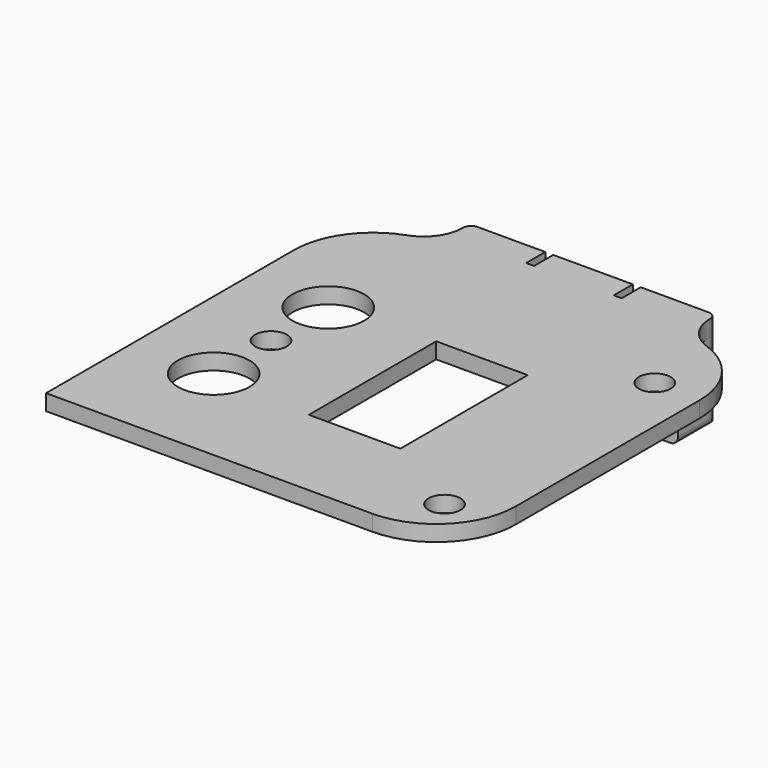
from build123d import *

# Parameters (mm, degrees)
F0_W     = 51
F0_H     = 48
F0_R     = 4.5
F0_R_2   = 2
F0_W_2   = 11.5
F0_H_2   = 20
F1_DEPTH = 2
F3_DEPTH = 6
F4_W     = 1
F4_H     = 12
F5_DEPTH = 3
F6_R     = 5
F7_R     = 0.99999
F8_R     = 10


# Not quite as in the source:
# - a fillet or chamfer is up to 0.001 mm smaller than in the source, because OpenCascade refuses the exact size


with BuildPart() as f1:
    # F0 (on Top) → F1 (new body)
    with BuildSketch(Plane.XY):
        with Locations((25.5, 24)):
            Rectangle(F0_W, F0_H)
        with Locations((10.25, 13.5)):
            Circle(F0_R, mode=Mode.SUBTRACT)
        with Locations((10.25, 22.5)):
            Circle(F0_R_2, mode=Mode.SUBTRACT)
        with Locations((45.25, 6)):
            Circle(F0_R_2, mode=Mode.SUBTRACT)
        with Locations((28.75, 22.5)):
            Rectangle(F0_W_2, F0_H_2, mode=Mode.SUBTRACT)
        with Locations((10.25, 31.5)):
            Circle(F0_R, mode=Mode.SUBTRACT)
        with Locations((45.25, 39)):
            Circle(F0_R_2, mode=Mode.SUBTRACT)
    extrude(amount=F1_DEPTH)

    # F2 (on face) → F3 (join)
    with BuildSketch(Plane(origin=(0, 48, 0), x_dir=(-1, 0, 0), z_dir=(0, 1, 0))):
        Polygon((-10, 2), (-41, 2), (-41, 0), (-41, -10), (-10, -10), (-10, 0), align=None)
    extrude(amount=F3_DEPTH)

    # F4 (on face) → F5 (cut)
    with BuildSketch(Plane(origin=(0, 54, 0), x_dir=(-1, 0, 0), z_dir=(0, 1, 0))):
        with Locations((-20, -4)):
            Rectangle(F4_W, F4_H)
        with Locations((-31, -4)):
            Rectangle(F4_W, F4_H)
    extrude(amount=-F5_DEPTH, mode=Mode.SUBTRACT)

    # F6
    f6_edges = [f1.edges().sort_by_distance(p)[0] for p in [
        (10, 48, 1),
        (41, 48, 1),
    ]]
    fillet(f6_edges, radius=F6_R)

    # F7 (radius 1 in the source; OpenCascade refuses exactly that, so slightly less here)
    f7_edges = [f1.edges().sort_by_distance(p)[0] for p in [
        (41, 54, -4),
        (10, 54, -4),
        (10, 51, -10),
        (41, 51, -10),
    ]]
    fillet(f7_edges, radius=F7_R)

    # F8
    f8_edges = [f1.edges().sort_by_distance(p)[0] for p in [
        (51, 48, 1),
        (0, 48, 1),
        (51, 0, 1),
    ]]
    fillet(f8_edges, radius=F8_R)


solid = f1.part
